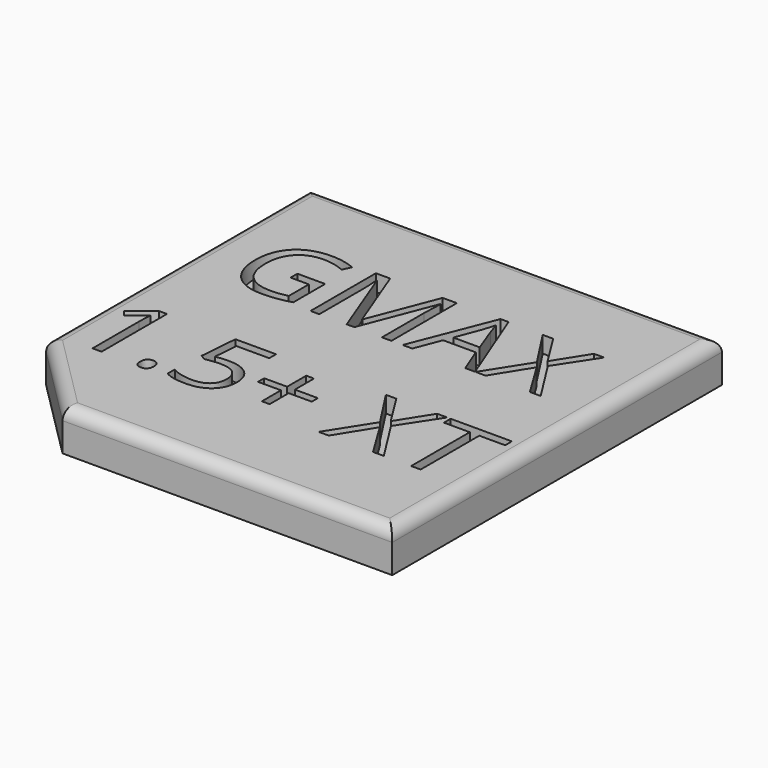
from build123d import *

# Parameters (mm, degrees)
F0_W         = 50
F0_H         = 50
F1_DEPTH     = 5
F2_TEXT_SIZE = 13.8888888889
F3_DEPTH     = 2
F4_SIZE      = 10
F5_R         = 1.5


# Not quite as in the source:
# - Text() gives the source's letters only with a copy of the font that has no kerning and outlines rounded to 1/6400 em; it was checked with that copy


with BuildPart() as f1:
    # F0 (on Top) → F1 (new body)
    with BuildSketch(Plane.XY):
        Rectangle(F0_W, F0_H)
    extrude(amount=F1_DEPTH)

    # F2 (on face) → F3 (cut)
    with BuildSketch(Plane.XY.offset(5)):
        with Locations((-20.3910590278, 5)):
            Text('GMAX', F2_TEXT_SIZE, font='Open Sans', text_align=(TextAlign.LEFT, TextAlign.BOTTOM))
        with Locations((-24, -13.8888888889)):
            Text('1.5+ XT', F2_TEXT_SIZE, font='Open Sans', text_align=(TextAlign.LEFT, TextAlign.BOTTOM))
    extrude(amount=-F3_DEPTH, mode=Mode.SUBTRACT)

    # F4
    f4_edges = [f1.edges().sort_by_distance(p)[0] for p in [
        (-25, -25, 2.5),
    ]]
    chamfer(f4_edges, length=F4_SIZE)

    # F5
    f5_edges = [f1.edges().sort_by_distance(p)[0] for p in [
        (5, -25, 5),
        (25, 0, 5),
        (0, 25, 5),
        (-25, 5, 5),
        (-20, -20, 5),
    ]]
    fillet(f5_edges, radius=F5_R)


solid = f1.part
